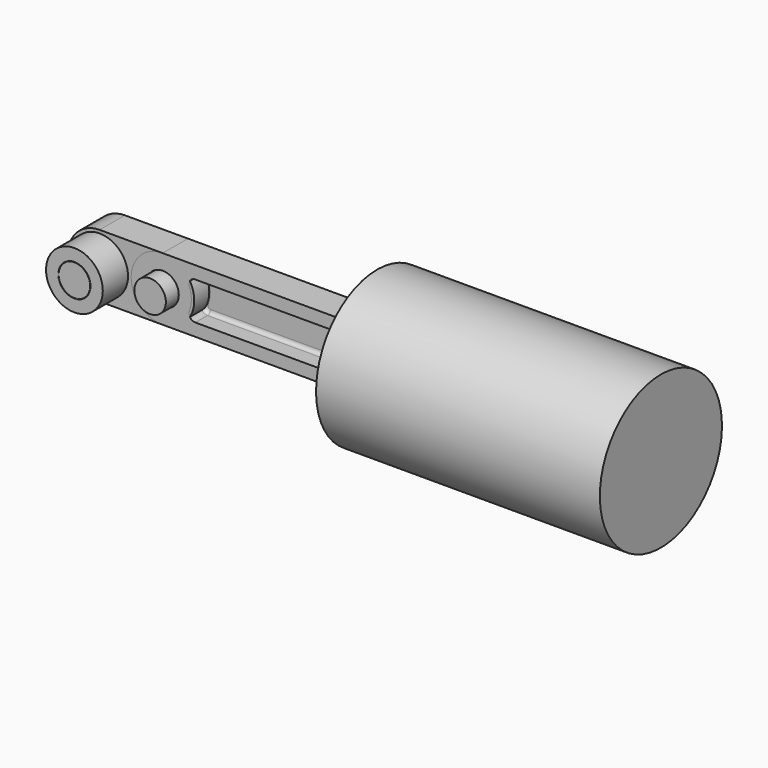
from build123d import *

# Parameters (mm, degrees)
F4_W      = 57.15
F4_H      = 2.54
F3_R      = 3.175
F6_DEPTH  = 6.35
F0_R      = 3.2385
F7_DEPTH  = 3.175
F1_R      = 3.2385
F24_DEPTH = 3.175
F9_R      = 3.2385
F10_DEPTH = 11.43
F12_R     = 3.175
F13_DEPTH = 11.43
F14_SIZE  = 1.27
F15_T     = -2.54
F16_R     = 1.27
F17_R     = 0.762
F18_R     = 3.175
F19_DEPTH = 6.35
F20_R     = 5.715
F20_R_2   = 3.2385
F21_DEPTH = 6.35
F22_R     = 12.827
F23_DEPTH = 2.54


with BuildPart() as f5:
    # F4 (on Front) → F5 (revolve)
    with BuildSketch(Plane.XZ):
        with Locations((81.915, 14.097)):
            Rectangle(F4_W, F4_H)
    revolve(axis=Axis((44.45, 0, 0), (1, 0, 0)))

    # F22 (on face) → F23 (join)
    with BuildSketch(Plane.YZ.offset(110.49)):
        Circle(F22_R)
    extrude(amount=-F23_DEPTH)


with BuildPart() as f6:
    # F3 (on Front) → F6 (new body, symmetric)
    with BuildSketch(Plane.XZ):
        with Locations((12.7, 0)):
            Circle(F3_R)
    extrude(amount=F6_DEPTH, both=True)


with BuildPart() as f7:
    # F0 (on Front) → F7 (new body, symmetric)
    with BuildSketch(Plane.XZ):
        with BuildLine():
            Line((12.7, 6.35), (0, 6.35))
            ThreePointArc((0, 6.35), (-6.35, 0), (0, -6.35))
            Line((0, -6.35), (12.7, -6.35))
            ThreePointArc((12.7, -6.35), (19.05, 0), (12.7, 6.35))
        make_face()
        with Locations((12.7, 0)):
            Circle(F0_R, mode=Mode.SUBTRACT)
    extrude(amount=F7_DEPTH, both=True)

    # F18 (on face) → F19 (join)
    with BuildSketch(Plane.XZ.offset(3.175)):
        Circle(F18_R)
    extrude(amount=F19_DEPTH)


with BuildPart() as f24:
    # F1 (on Front) → F24 (new body, symmetric)
    with BuildSketch(Plane.XZ):
        with BuildLine():
            Line((88.9, 6.35), (12.7, 6.35))
            ThreePointArc((12.7, 6.35), (6.35, 0), (12.7, -6.35))
            Line((12.7, -6.35), (88.9, -6.35))
            ThreePointArc((88.9, -6.35), (95.25, 0), (88.9, 6.35))
        make_face()
        with Locations((12.7, 0)):
            Circle(F1_R, mode=Mode.SUBTRACT)
        with Locations((88.9, 0)):
            Circle(F1_R, mode=Mode.SUBTRACT)
    extrude(amount=F24_DEPTH, both=True)

    # F15
    f15_openings = [f24.faces().sort_by_distance(p)[0] for p in [
        (50.8, -3.175, 0),
    ]]
    offset(amount=F15_T, openings=f15_openings, kind=Kind.INTERSECTION)

    # F16
    f16_edges = [f24.edges().sort_by_distance(p)[0] for p in [
        (84.555468, -1.27, -3.81),
        (17.044532, -1.27, -3.81),
        (84.555468, -1.27, 3.81),
        (17.044532, -1.27, 3.81),
    ]]
    fillet(f16_edges, radius=F16_R)

    # F17
    f17_edges = [f24.edges().sort_by_distance(p)[0] for p in [
        (50.8, 0.635, -3.81),
        (83.372474, 0.635, -3.258218),
        (18.227526, 0.635, -3.258218),
        (83.1215, 0.635, 0),
        (18.380611, 0.635, -1.059113),
        (83.372474, 0.635, 3.258218),
        (18.380611, 0.635, 1.059113),
        (50.8, 0.635, 3.81),
        (18.227526, 0.635, 3.258218),
    ]]
    fillet(f17_edges, radius=F17_R)


with BuildPart() as f8:
    # F2 (on Front) → F8 (revolve)
    with BuildSketch(Plane.XZ):
        Polygon((107.95, 12.7), (82.55, 12.7), (82.55, 10.16), (104.14, 10.16), (104.14, 0), (107.95, 0), align=None)
    revolve(axis=Axis((44.45, 0, 0), (1, 0, 0)))


with BuildPart() as f10:
    # F9 (on Front) → F10 (new body, symmetric)
    with BuildSketch(Plane.XZ):
        with Locations((88.9, 0)):
            Circle(F9_R)
    extrude(amount=F10_DEPTH, both=True)


with BuildPart() as f8_1:
    add(f8.part)

    # F11: cut F10
    add(f10.part, mode=Mode.SUBTRACT)

    # F14
    f14_edges = [f8_1.edges().sort_by_distance(p)[0] for p in [
        (107.95, 0, -12.7),
        (82.55, 0, -12.7),
    ]]
    chamfer(f14_edges, length=F14_SIZE)


with BuildPart() as f13:
    # F12 (on Front) → F13 (new body, symmetric)
    with BuildSketch(Plane.XZ):
        with Locations((88.9, 0)):
            Circle(F12_R)
    extrude(amount=F13_DEPTH, both=True)


with BuildPart() as f21:
    # F20 (on face) → F21 (new body)
    with BuildSketch(Plane.XZ.offset(3.175)):
        Circle(F20_R)
        Circle(F20_R_2, mode=Mode.SUBTRACT)
    extrude(amount=F21_DEPTH)


solid = Compound([f5.part, f6.part, f7.part, f24.part, f8_1.part, f13.part, f21.part])
